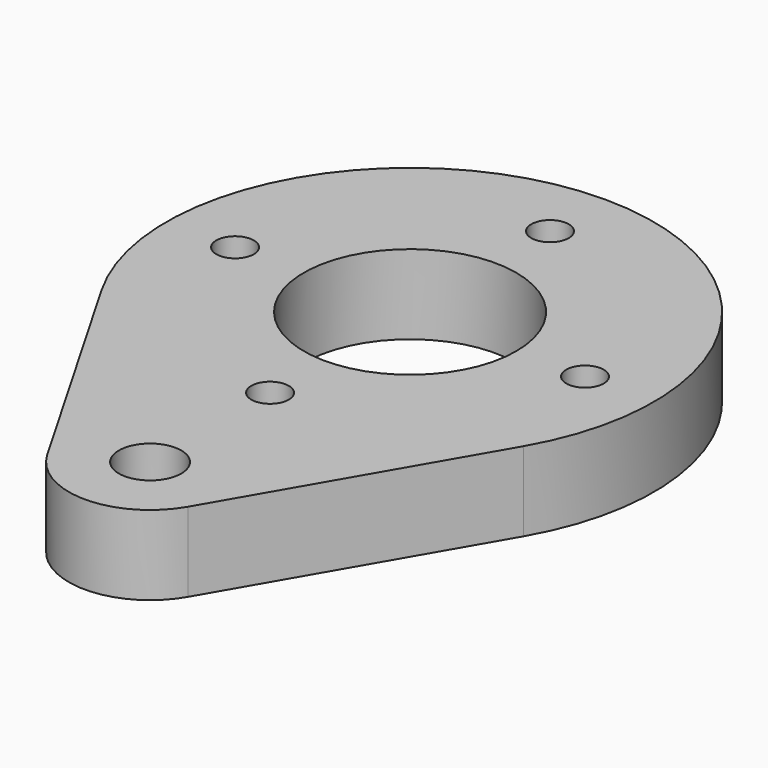
from build123d import *

# Parameters (mm, degrees)
F0_R     = 1.25
F0_R_2   = 0.75
F0_R_3   = 4.25
F1_DEPTH = 3.175


# Not quite as in the source:
# - a length typed as a fraction of an inch, garbled in the dataset ("3 / 203.2 mm" for 3/8 in), is restored


with BuildPart() as f1:
    # F0 (on Top) → F1 (new body)
    with BuildSketch(Plane.XY):
        with BuildLine():
            Line((-38.4956756474, 4.4767191038), (-32.8665105228, 14.2267191038))
            ThreePointArc((-32.8665105228, 14.2267191038), (-41.3102582097, 28.8517191038), (-49.7540058966, 14.2267191038))
            Line((-49.7540058966, 14.2267191038), (-44.124840772, 4.4767191038))
            ThreePointArc((-44.124840772, 4.4767191038), (-41.3102582097, 2.8517191038), (-38.4956756474, 4.4767191038))
        make_face()
        with Locations((-41.3102582097, 6.1017191038)):
            Circle(F0_R, mode=Mode.SUBTRACT)
        with Locations((-41.3102582097, 12.1017191038)):
            Circle(F0_R_2, mode=Mode.SUBTRACT)
        with Locations((-48.3102582097, 19.1017191038)):
            Circle(F0_R_2, mode=Mode.SUBTRACT)
        with Locations((-41.3102582097, 19.1017191038)):
            Circle(F0_R_3, mode=Mode.SUBTRACT)
        with Locations((-34.3102582097, 19.1017191038)):
            Circle(F0_R_2, mode=Mode.SUBTRACT)
        with Locations((-41.3102582097, 26.1017191038)):
            Circle(F0_R_2, mode=Mode.SUBTRACT)
    extrude(amount=F1_DEPTH)


solid = f1.part
